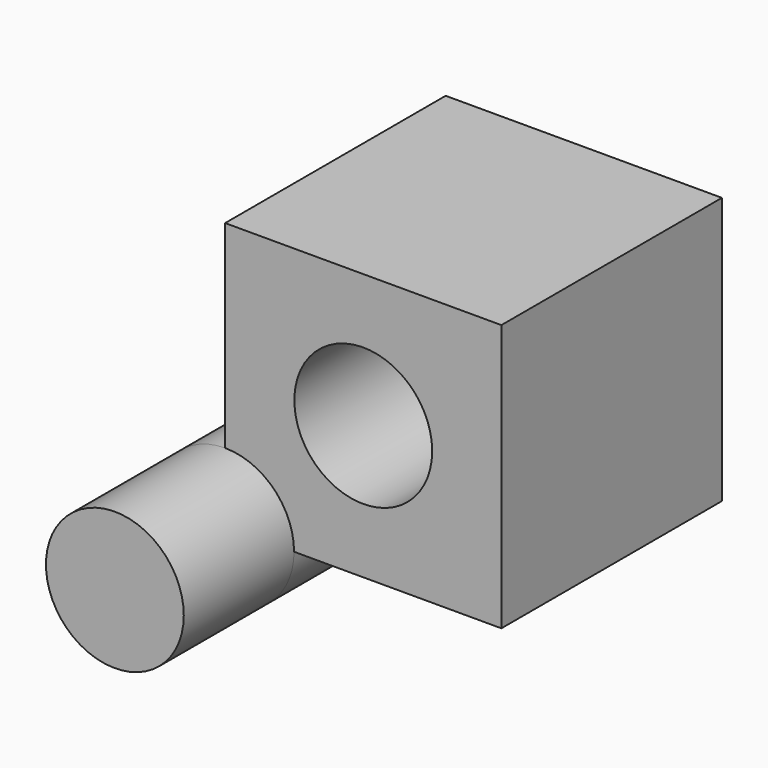
from build123d import *

# Parameters (mm, degrees)
F0_W          = 101.8202751875
F0_H          = 98.3881354332
F0_R          = 25.4
F1_DEPTH      = 101.6
F4_R          = 25.4
F5_DEPTH      = 50.8
F5_DEPTH_BACK = 152.4


# Not quite as in the source:
# - a feature of the source that left no trace in its solid (it failed there, or was rolled back) is left out


with BuildPart() as f1:
    # F0 (on Front) → F1 (new body)
    with BuildSketch(Plane.XZ):
        with Locations((50.9101375937, 49.1940677166)):
            Rectangle(F0_W, F0_H)
        with Locations((50.9101375937, 49.1940677166)):
            Circle(F0_R, mode=Mode.SUBTRACT)
    extrude(amount=F1_DEPTH)

    # F4 (on offset) → F5 (join, two sides)
    with BuildSketch(Plane.XZ.offset(101.6)) as f5_sk:
        Circle(F4_R)
    extrude(amount=F5_DEPTH)
    extrude(f5_sk.sketch, amount=-F5_DEPTH_BACK)


solid = f1.part
